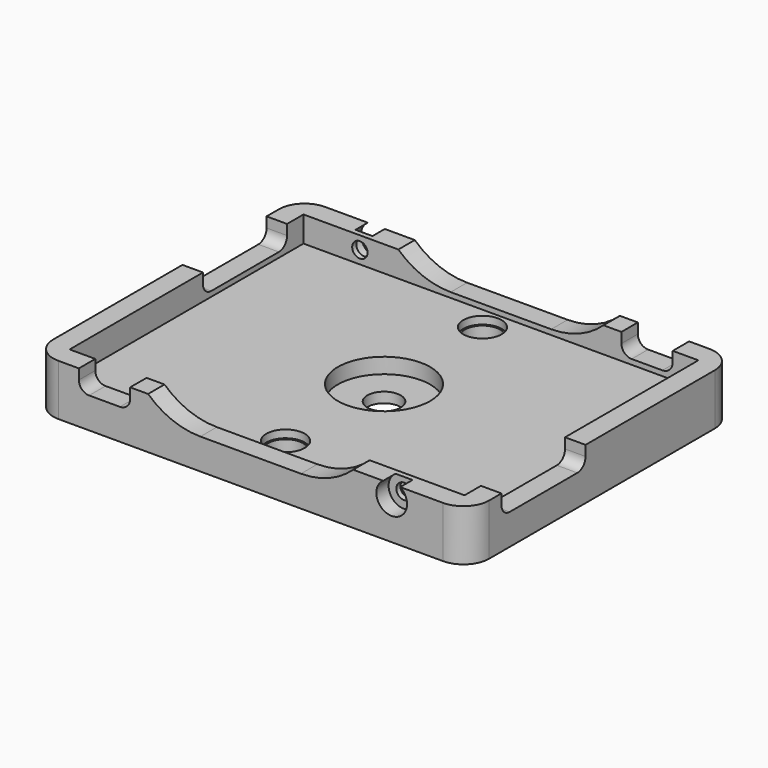
from build123d import *

# Parameters (mm, degrees)
F0_W                   = 85
F0_H                   = 65
F0_W_2                 = 77
F0_H_2                 = 57
F1_DEPTH               = 5
F2_DEPTH               = 5
F3_W                   = 10
F3_H                   = 4
F3_W_2                 = 40
F3_W_3                 = 4
F3_H_2                 = 20.5
F4_DEPTH               = 4
F5_T1_DEPTH            = 4
F5_T3_DEPTH            = 4
F6_R                   = 2
F8_D                   = 6.8
F8_CBORE_D             = 7.5
F8_CBORE_DEPTH         = 1.5
F9_R                   = 9
F9_R_2                 = 3.25
F10_DEPTH              = 3
F11_DEPTH              = 25
F12_R                  = 5
F15_D                  = 3
F15_CBORE_D            = 6
F15_CBORE_DEPTH        = 3
F15_ON_F13_D           = 3
F15_ON_F13_CBORE_D     = 6
F15_ON_F13_CBORE_DEPTH = 3


# Not quite as in the source:
# - a fillet or chamfer that OpenCascade refuses, or shapes differently, is made with other operations: its cross-section is extruded or revolved along the edge and cut away or added


with BuildPart() as f1:
    # F0 (on Top) → F1 (new body)
    with BuildSketch(Plane.XY):
        Rectangle(F0_W, F0_H)
        Rectangle(F0_W_2, F0_H_2, mode=Mode.SUBTRACT)
        Rectangle(F0_W_2, F0_H_2)
    extrude(amount=-F1_DEPTH)

    # F0 (on Top) → F2 (join)
    with BuildSketch(Plane.XY):
        Rectangle(F0_W, F0_H)
        Rectangle(F0_W_2, F0_H_2, mode=Mode.SUBTRACT)
    extrude(amount=F2_DEPTH)

    # F3 (on face) → F4 (cut)
    with BuildSketch(Plane.XY.offset(5)):
        with Locations((28.5, 30.5)):
            Rectangle(F3_W, F3_H)
        with Locations((0, 30.5)):
            Rectangle(F3_W_2, F3_H)
        with Locations((0, -30.5)):
            Rectangle(F3_W_2, F3_H)
        with Locations((-28.5, -30.5)):
            Rectangle(F3_W, F3_H)
        with Locations((-40.5, 14.25)):
            Rectangle(F3_W_3, F3_H_2)
        with Locations((40.5, -14.25)):
            Rectangle(F3_W_3, F3_H_2)
    extrude(amount=-F4_DEPTH, mode=Mode.SUBTRACT)

    # F5: fillet of radius 15 on 4 edges, made by hand

    # F5_s2 → F5_t1 (join)
    with BuildSketch(Plane.XZ.offset(-32.5)):
        with BuildLine():
            ThreePointArc((-9.8019609728, 1), (-15.2791865479, 2.0357599562), (-20, 5))
            Line((-20, 5), (-20, 1))
            Line((-20, 1), (-9.8019609728, 1))
        make_face()
        with BuildLine():
            ThreePointArc((20, 5), (15.2791865479, 2.0357599562), (9.8019609728, 1))
            Line((9.8019609728, 1), (20, 1))
            Line((20, 1), (20, 5))
        make_face()
    extrude(amount=F5_T1_DEPTH)

    # F5_s4 → F5_t3 (join)
    with BuildSketch(Plane.XZ.offset(28.5)):
        with BuildLine():
            ThreePointArc((9.8019609728, 1), (15.2791865479, 2.0357599562), (20, 5))
            Line((20, 5), (20, 1))
            Line((20, 1), (9.8019609728, 1))
        make_face()
        with BuildLine():
            ThreePointArc((-20, 5), (-15.2791865479, 2.0357599562), (-9.8019609728, 1))
            Line((-9.8019609728, 1), (-20, 1))
            Line((-20, 1), (-20, 5))
        make_face()
    extrude(amount=F5_T3_DEPTH)

    # F6
    f6_edges = [f1.edges().sort_by_distance(p)[0] for p in [
        (40.5, -4, 1),
        (40.5, -24.5, 1),
        (-40.5, 24.5, 1),
        (-40.5, 4, 1),
        (-33.5, -30.5, 1),
        (-23.5, -30.5, 1),
        (33.5, 30.5, 1),
        (23.5, 30.5, 1),
    ]]
    fillet(f6_edges, radius=F6_R)

    # F8 (through all)
    with Locations(Plane.XY):
        with Locations((0, 24), (0, -24)):
            CounterBoreHole(F8_D / 2, F8_CBORE_D / 2, F8_CBORE_DEPTH)

    # F9 (on face) → F10 (cut)
    with BuildSketch(Plane.XY):
        Circle(F9_R)
        Circle(F9_R_2, mode=Mode.SUBTRACT)
    extrude(amount=-F10_DEPTH, mode=Mode.SUBTRACT)

    # F9 (on face) → F11 (cut)
    with BuildSketch(Plane.XY):
        Circle(F9_R_2)
    extrude(amount=-F11_DEPTH, mode=Mode.SUBTRACT)

    # F12
    f12_edges = [f1.edges().sort_by_distance(p)[0] for p in [
        (42.5, -32.5, 0),
        (42.5, 32.5, 0),
        (-42.5, -32.5, 0),
        (-42.5, 32.5, 0),
    ]]
    fillet(f12_edges, radius=F12_R)

    # F15 (through all)
    with Locations(Plane(origin=(0, 32.5, 0), x_dir=(-1, 0, 0), z_dir=(0, 1, 0))):
        with Locations((27.5, 2.5)):
            CounterBoreHole(F15_D / 2, F15_CBORE_D / 2, F15_CBORE_DEPTH)

    # F15 on F13 (through all)
    with Locations(Plane.XZ.offset(32.5)):
        with Locations((27.5, 2.5)):
            CounterBoreHole(F15_ON_F13_D / 2, F15_ON_F13_CBORE_D / 2, F15_ON_F13_CBORE_DEPTH)


solid = f1.part
